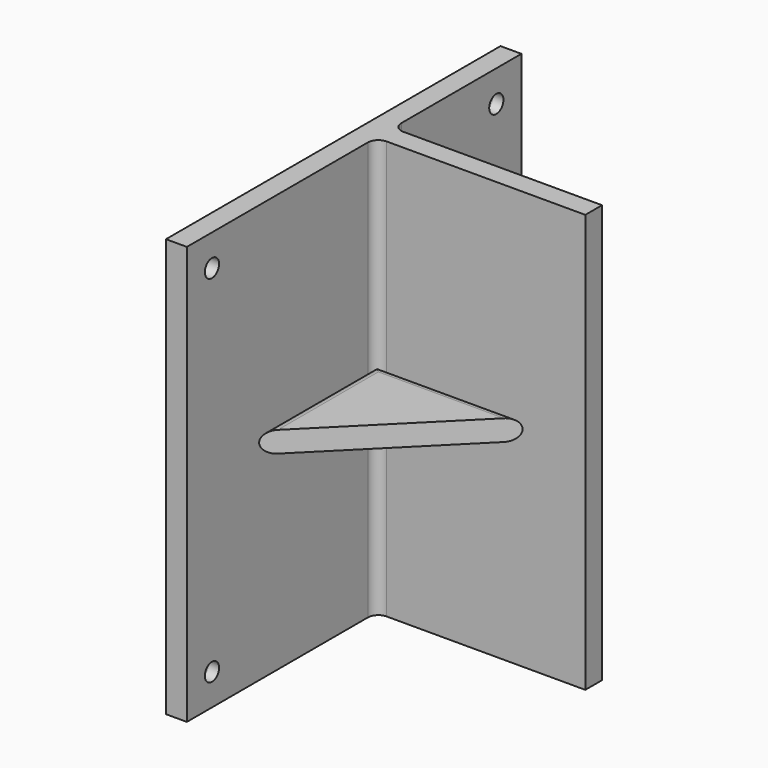
from build123d import *

# Parameters (mm, degrees)
F0_W      = 100
F0_H      = 10
F1_DEPTH  = 200
F2_W      = 70
F2_H      = 10
F3_DEPTH  = 70
F5_DEPTH  = 70
F6_R      = 4.25
F7_DEPTH  = 12.5
F9_W      = 70
F9_H      = 10
F10_DEPTH = 70
F12_DEPTH = 25
F13_R     = 4.99999
F13_2_R   = 4.99999


# Not quite as in the source:
# - a fillet or chamfer is up to 0.001 mm smaller than in the source, because OpenCascade refuses the exact size


with BuildPart() as f1:
    # F0 (on Top) → F1 (new body)
    with BuildSketch(Plane.XY):
        Polygon((5, 100), (-5, 100), (-5, -100), (5, -100), (5, 13.2), (5, 23.2), align=None)
        with Locations((55, 18.2)):
            Rectangle(F0_W, F0_H)
    extrude(amount=F1_DEPTH)

    # F6 (on Right) → F7 (cut, symmetric)
    with BuildSketch(Plane.YZ):
        with Locations((85, 185)):
            Circle(F6_R)
        with Locations((85, 15)):
            Circle(F6_R)
        with Locations((-85, 15)):
            Circle(F6_R)
        with Locations((-85, 185)):
            Circle(F6_R)
    extrude(amount=F7_DEPTH, both=True, mode=Mode.SUBTRACT)

    # F13 (radius 5 in the source; OpenCascade refuses exactly that, so slightly less here)
    f13_edges = [f1.edges().sort_by_distance(p)[0] for p in [
        (5, 13.2, 100),
        (5, 23.2, 100),
    ]]
    fillet(f13_edges, radius=F13_R)


with BuildPart() as f3:
    # F2 (on face) → F3 (new body)
    with BuildSketch(Plane.YZ.offset(5)):
        with Locations((-21.8, 100)):
            Rectangle(F2_W, F2_H)
    extrude(amount=F3_DEPTH)

    # F4 (on face) → F5 (cut)
    with BuildSketch(Plane.XY.offset(105)):
        Polygon((75, 13.2), (5, -56.8), (75, -56.8), align=None)
    extrude(amount=-F5_DEPTH, mode=Mode.SUBTRACT)


with BuildPart() as f10:
    # F9 (on face) → F10 (new body)
    with BuildSketch(Plane.YZ.offset(5)):
        with Locations((-21.8, 100)):
            Rectangle(F9_W, F9_H)
    extrude(amount=F10_DEPTH)

    # F11 (on face) → F12 (cut)
    with BuildSketch(Plane.XY.offset(105)):
        Polygon((75, 13.2), (5, -56.8), (75, -56.8), align=None)
    extrude(amount=-F12_DEPTH, mode=Mode.SUBTRACT)

    # F13#2 (radius 5 in the source; OpenCascade refuses exactly that, so slightly less here)
    f13_2_edges = [f10.edges().sort_by_distance(p)[0] for p in [
        (40, 13.2, 105),
        (5, -21.8, 105),
        (5, -21.8, 95),
        (40, 13.2, 95),
    ]]
    fillet(f13_2_edges, radius=F13_2_R)


solid = Compound([f1.part, f10.part])
